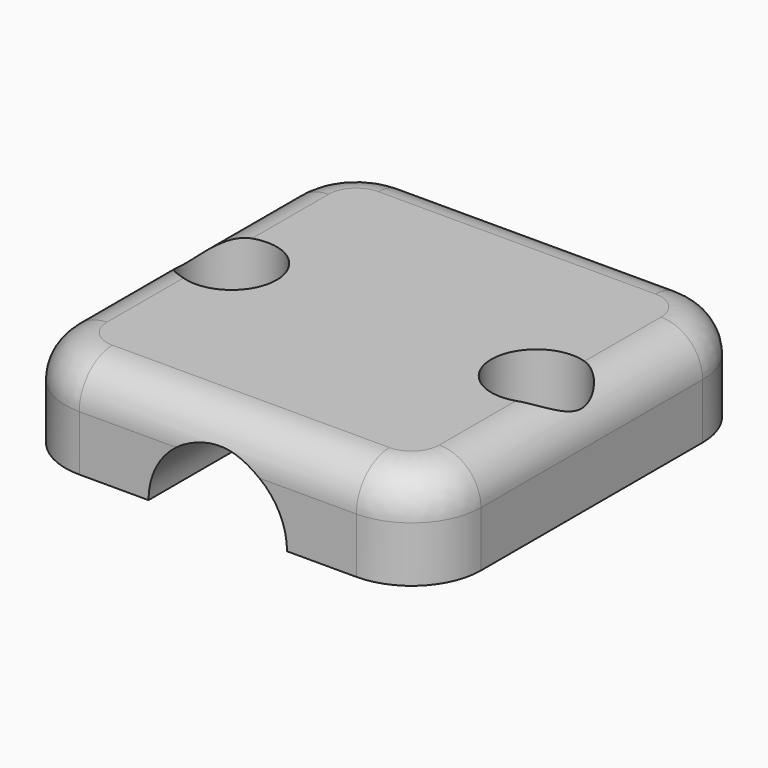
from build123d import *

# Parameters (mm, degrees)
F0_W           = 30
F0_H           = 30
F1_DEPTH       = 7
F3_D           = 3.4
F3_CBORE_D     = 6.5
F3_CBORE_DEPTH = 4
F5_DEPTH       = 30
F6_R           = 5
F7_T1_DEPTH    = 20
F7_T3_DEPTH    = 20
F7_T6_ANGLE    = 90
F7_T8_ANGLE    = 90
F7_T10_ANGLE   = 90
F7_T12_ANGLE   = 90


# Not quite as in the source:
# - a fillet or chamfer that OpenCascade refuses, or shapes differently, is made with other operations: its cross-section is extruded or revolved along the edge and cut away or added


with BuildPart() as f1:
    # F0 (on Top) → F1 (new body)
    with BuildSketch(Plane.XY):
        Rectangle(F0_W, F0_H)
    extrude(amount=F1_DEPTH)

    # F3 (through all)
    with Locations(Plane.XY.offset(7)):
        with Locations((-11, 0), (11, 0)):
            CounterBoreHole(F3_D / 2, F3_CBORE_D / 2, F3_CBORE_DEPTH)

    # F4 (on face) → F5 (cut, through all)
    with BuildSketch(Plane.XZ.offset(15)):
        with BuildLine():
            Line((-5, 0), (5, 0))
            ThreePointArc((5, 0), (0, 5), (-5, 0))
        make_face()
    extrude(amount=-F5_DEPTH, mode=Mode.SUBTRACT)

    # F6
    f6_edges = [f1.edges().sort_by_distance(p)[0] for p in [
        (15, -15, 3.5),
        (-15, -15, 3.5),
        (15, 15, 3.5),
        (-15, 15, 3.5),
    ]]
    fillet(f6_edges, radius=F6_R)

    # F7: fillet of radius 3 on 8 edges, made by hand

    # F7_s2 → F7_t1 (cut)
    with BuildSketch(Plane.YZ.offset(-10)):
        with BuildLine():
            ThreePointArc((-15, 4), (-14.1213203436, 6.1213203436), (-12, 7))
            Line((-12, 7), (-15, 7))
            Line((-15, 7), (-15, 4))
        make_face()
        with BuildLine():
            ThreePointArc((12, 7), (14.1213203436, 6.1213203436), (15, 4))
            Line((15, 4), (15, 7))
            Line((15, 7), (12, 7))
        make_face()
    extrude(amount=F7_T1_DEPTH, mode=Mode.SUBTRACT)

    # F7_s4 → F7_t3 (cut)
    with BuildSketch(Plane.XZ.offset(-10)):
        with BuildLine():
            ThreePointArc((-12, 7), (-14.1213203436, 6.1213203436), (-15, 4))
            Line((-15, 4), (-15, 7))
            Line((-15, 7), (-12, 7))
        make_face()
        with BuildLine():
            ThreePointArc((12, 7), (14.1213203436, 6.1213203436), (15, 4))
            Line((15, 4), (15, 7))
            Line((15, 7), (12, 7))
        make_face()
    extrude(amount=F7_T3_DEPTH, mode=Mode.SUBTRACT)

    # F7_s5 → F7_t6 (revolve, cut)
    with BuildSketch(Plane.YZ.offset(-10)):
        with BuildLine():
            ThreePointArc((-15, 4), (-14.1213203436, 6.1213203436), (-12, 7))
            Line((-12, 7), (-15, 7))
            Line((-15, 7), (-15, 4))
        make_face()
    revolve(axis=Axis((-10, -10, 7), (0, 0, -1)), revolution_arc=F7_T6_ANGLE, mode=Mode.SUBTRACT)

    # F7_s7 → F7_t8 (revolve, cut)
    with BuildSketch(Plane.YZ.offset(10)):
        with BuildLine():
            ThreePointArc((-12, 7), (-14.1213203436, 6.1213203436), (-15, 4))
            Line((-15, 4), (-15, 7))
            Line((-15, 7), (-12, 7))
        make_face()
    revolve(axis=Axis((10, -10, 7), (0, 0, 1)), revolution_arc=F7_T8_ANGLE, mode=Mode.SUBTRACT)

    # F7_s9 → F7_t10 (revolve, cut)
    with BuildSketch(Plane.XZ.offset(-10)):
        with BuildLine():
            ThreePointArc((-12, 7), (-14.1213203436, 6.1213203436), (-15, 4))
            Line((-15, 4), (-15, 7))
            Line((-15, 7), (-12, 7))
        make_face()
    revolve(axis=Axis((-10, 10, 7), (0, 0, -1)), revolution_arc=F7_T10_ANGLE, mode=Mode.SUBTRACT)

    # F7_s11 → F7_t12 (revolve, cut)
    with BuildSketch(Plane.XZ.offset(-10)):
        with BuildLine():
            ThreePointArc((12, 7), (14.1213203436, 6.1213203436), (15, 4))
            Line((15, 4), (15, 7))
            Line((15, 7), (12, 7))
        make_face()
    revolve(axis=Axis((10, 10, 7), (0, 0, 1)), revolution_arc=F7_T12_ANGLE, mode=Mode.SUBTRACT)


solid = f1.part
